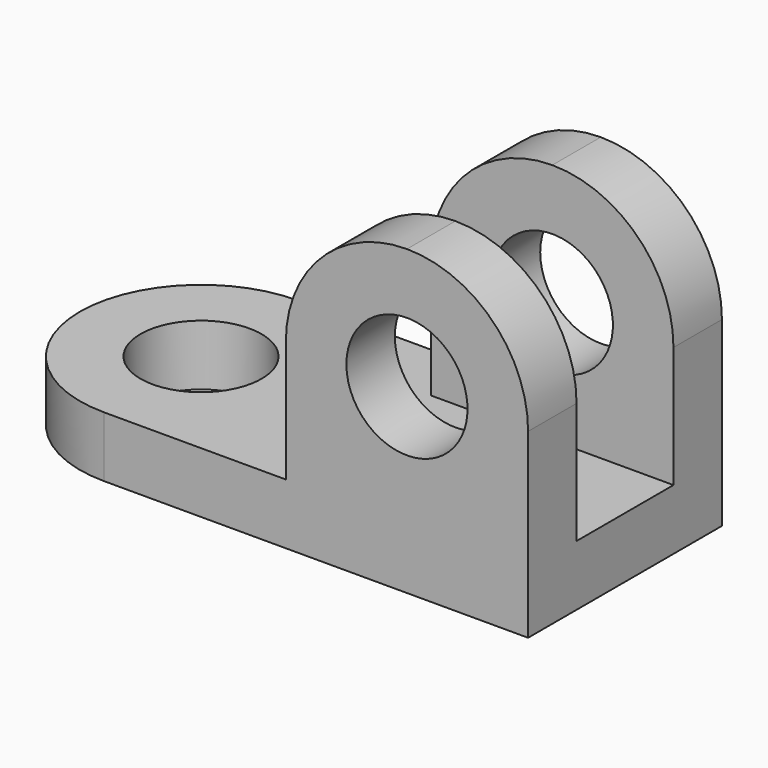
from build123d import *

# Parameters (mm, degrees)
F1_DEPTH = 12.7
F2_W     = 50.8
F2_H     = 12.7
F3_DEPTH = 50.8
F4_D     = 25.4
F5_R     = 25.4
F6_R     = 25.39999
F7_R     = 25.4
F8_R     = 25.39999
F10_D    = 25.4


# Not quite as in the source:
# - a fillet or chamfer is up to 0.001 mm smaller than in the source, because OpenCascade refuses the exact size


with BuildPart() as f1:
    # F0 (on Top) → F1 (new body)
    with BuildSketch(Plane.XY):
        with BuildLine():
            ThreePointArc((0, 25.4), (7.4394877579, 7.4394877579), (25.4, 0))
            Line((25.4, 0), (114.3, 0))
            Line((114.3, 0), (114.3, 50.8))
            Line((114.3, 50.8), (25.4, 50.8))
            ThreePointArc((25.4, 50.8), (7.4394877579, 43.3605122421), (0, 25.4))
        make_face()
    extrude(amount=F1_DEPTH)

    # F2 (on face) → F3 (join)
    with BuildSketch(Plane.XY.offset(12.7)):
        with Locations((88.9, 6.35)):
            Rectangle(F2_W, F2_H)
        with Locations((88.9, 44.45)):
            Rectangle(F2_W, F2_H)
    extrude(amount=F3_DEPTH)

    # F4 (through all)
    with Locations(Plane.XY.offset(12.7)):
        with Locations((25.4, 25.4)):
            Hole(F4_D / 2)

    # F5
    f5_edges = [f1.edges().sort_by_distance(p)[0] for p in [
        (63.5, 6.35, 63.5),
    ]]
    fillet(f5_edges, radius=F5_R)

    # F6 (radius 25.4 in the source; OpenCascade refuses exactly that, so slightly less here)
    f6_edges = [f1.edges().sort_by_distance(p)[0] for p in [
        (114.3, 6.35, 63.5),
    ]]
    fillet(f6_edges, radius=F6_R)

    # F7
    f7_edges = [f1.edges().sort_by_distance(p)[0] for p in [
        (63.5, 44.45, 63.5),
    ]]
    fillet(f7_edges, radius=F7_R)

    # F8 (radius 25.4 in the source; OpenCascade refuses exactly that, so slightly less here)
    f8_edges = [f1.edges().sort_by_distance(p)[0] for p in [
        (114.3, 44.45, 63.5),
    ]]
    fillet(f8_edges, radius=F8_R)

    # F10 (through all)
    with Locations(Plane.XZ):
        with Locations((88.9, 38.1)):
            Hole(F10_D / 2)


solid = f1.part
